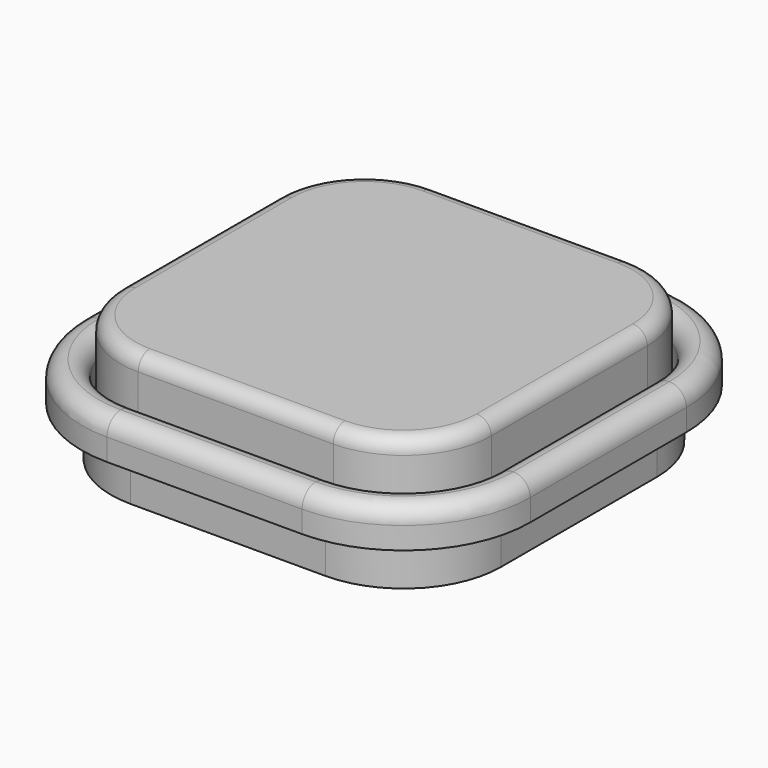
from build123d import *

# Parameters (mm, degrees)
F1_DEPTH = 2.5
F3_DEPTH = 2
F4_R     = 0.87499
F6_DEPTH = 4
F7_R     = 0.75


# Not quite as in the source:
# - a fillet or chamfer is up to 0.001 mm smaller than in the source, because OpenCascade refuses the exact size


with BuildPart() as f1:
    # F0 (on Top) → F1 (new body)
    with BuildSketch(Plane.XY):
        with BuildLine():
            Line((-5, -10), (5, -10))
            ThreePointArc((5, -10), (8.5355339059, -8.5355339059), (10, -5))
            Line((10, -5), (10, 5))
            ThreePointArc((10, 5), (8.5355339059, 8.5355339059), (5, 10))
            Line((5, 10), (-5, 10))
            ThreePointArc((-5, 10), (-8.5355339059, 8.5355339059), (-10, 5))
            Line((-10, 5), (-10, -5))
            ThreePointArc((-10, -5), (-8.5355339059, -8.5355339059), (-5, -10))
        make_face()
    extrude(amount=F1_DEPTH)

    # F2 (on face) → F3 (join)
    with BuildSketch(Plane.XY.offset(2.5)):
        with BuildLine():
            Line((-5, -11.5), (5, -11.5))
            ThreePointArc((5, -11.5), (9.5961940777, -9.5961940777), (11.5, -5))
            Line((11.5, -5), (11.5, 5))
            ThreePointArc((11.5, 5), (9.5961940777, 9.5961940777), (5, 11.5))
            Line((5, 11.5), (-5, 11.5))
            ThreePointArc((-5, 11.5), (-9.5961940777, 9.5961940777), (-11.5, 5))
            Line((-11.5, 5), (-11.5, -5))
            ThreePointArc((-11.5, -5), (-9.5961940777, -9.5961940777), (-5, -11.5))
        make_face()
        with BuildLine():
            ThreePointArc((9.75, -5), (8.3587572106, -8.3587572106), (5, -9.75))
            Line((5, -9.75), (-5, -9.75))
            ThreePointArc((-5, -9.75), (-8.3587572106, -8.3587572106), (-9.75, -5))
            Line((-9.75, -5), (-9.75, 5))
            ThreePointArc((-9.75, 5), (-8.3587572106, 8.3587572106), (-5, 9.75))
            Line((-5, 9.75), (5, 9.75))
            ThreePointArc((5, 9.75), (8.3587572106, 8.3587572106), (9.75, 5))
            Line((9.75, 5), (9.75, -5))
        make_face(mode=Mode.SUBTRACT)
    extrude(amount=F3_DEPTH)

    # F4 (radius 0.875 in the source; OpenCascade refuses exactly that, so slightly less here)
    f4_edges = [f1.edges().sort_by_distance(p)[0] for p in [
        (-9.75, 0, 4.5),
        (-11.5, 0, 4.5),
    ]]
    fillet(f4_edges, radius=F4_R)

    # F5 (on face) → F6 (join)
    with BuildSketch(Plane.XY.offset(2.5)):
        with BuildLine():
            ThreePointArc((9.5, 5), (8.1819805153, 8.1819805153), (5, 9.5))
            Line((5, 9.5), (-5, 9.5))
            ThreePointArc((-5, 9.5), (-8.1819805153, 8.1819805153), (-9.5, 5))
            Line((-9.5, 5), (-9.5, -5))
            ThreePointArc((-9.5, -5), (-8.1819805153, -8.1819805153), (-5, -9.5))
            Line((-5, -9.5), (5, -9.5))
            ThreePointArc((5, -9.5), (8.1819805153, -8.1819805153), (9.5, -5))
            Line((9.5, -5), (9.5, 5))
        make_face()
    extrude(amount=F6_DEPTH)

    # F7
    f7_edges = [f1.edges().sort_by_distance(p)[0] for p in [
        (0, -9.5, 6.5),
    ]]
    fillet(f7_edges, radius=F7_R)


solid = f1.part
